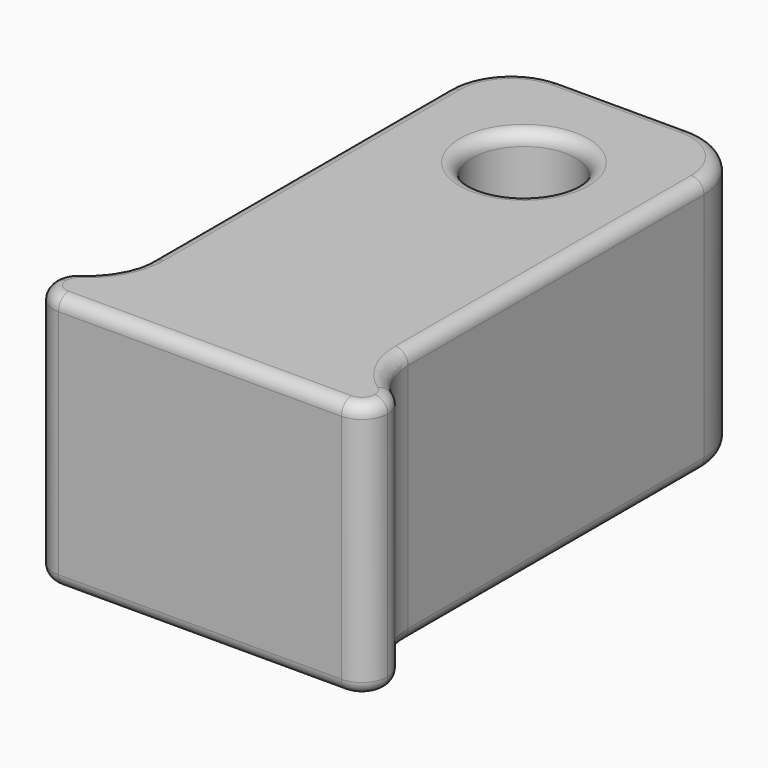
from build123d import *

# Parameters (mm, degrees)
F0_R     = 4
F1_DEPTH = 20
F2_R     = 5
F3_R     = 1.99999
F4_R     = 5
F5_R     = 1


# Not quite as in the source:
# - a fillet or chamfer is up to 0.001 mm smaller than in the source, because OpenCascade refuses the exact size


with BuildPart() as f1:
    # F0 (on Top) → F1 (new body)
    with BuildSketch(Plane.XY):
        Polygon((-10, -20.75), (10, -20.75), (13, -20.75), (13, -16.75), (10, -16.75), (10, 20.75), (-10, 20.75), (-10, -16.75), (-13, -16.75), (-13, -20.75), align=None)
        with Locations((0, 10.75)):
            Circle(F0_R, mode=Mode.SUBTRACT)
    extrude(amount=F1_DEPTH)

    # F2
    f2_edges = [f1.edges().sort_by_distance(p)[0] for p in [
        (-10, 20.75, 10),
        (10, 20.75, 10),
    ]]
    fillet(f2_edges, radius=F2_R)

    # F3 (radius 2 in the source; OpenCascade refuses exactly that, so slightly less here)
    f3_edges = [f1.edges().sort_by_distance(p)[0] for p in [
        (-13, -16.75, 10),
        (-13, -20.75, 10),
        (13, -16.75, 10),
        (13, -20.75, 10),
    ]]
    fillet(f3_edges, radius=F3_R)

    # F4
    f4_edges = [f1.edges().sort_by_distance(p)[0] for p in [
        (-10, -16.75, 10),
        (10, -16.75, 10),
    ]]
    fillet(f4_edges, radius=F4_R)

    # F5
    f5_edges = [f1.edges().sort_by_distance(p)[0] for p in [
        (12.772811, -17.824174, 20),
        (10.567975, -15.319984, 20),
        (13, -18.75, 20),
        (10, 1.372284, 20),
        (12.414216, -20.164216, 20),
        (8.535534, 19.285534, 20),
        (0, -20.75, 20),
        (0, 20.75, 20),
        (-12.414216, -20.164216, 20),
        (-8.535534, 19.285534, 20),
        (-13, -18.75, 20),
        (-10, 1.372284, 20),
        (-12.772811, -17.824174, 20),
        (-10.567975, -15.319984, 20),
        (-4, 10.75, 20),
        (12.772811, -17.824174, 0),
        (10.567975, -15.319984, 0),
        (13, -18.75, 0),
        (10, 1.372284, 0),
        (12.414216, -20.164216, 0),
        (8.535534, 19.285534, 0),
        (0, -20.75, 0),
        (0, 20.75, 0),
        (-12.414216, -20.164216, 0),
        (-8.535534, 19.285534, 0),
        (-13, -18.75, 0),
        (-10, 1.372284, 0),
        (-12.772811, -17.824174, 0),
        (-10.567975, -15.319984, 0),
        (-4, 10.75, 0),
    ]]
    fillet(f5_edges, radius=F5_R)


solid = f1.part
